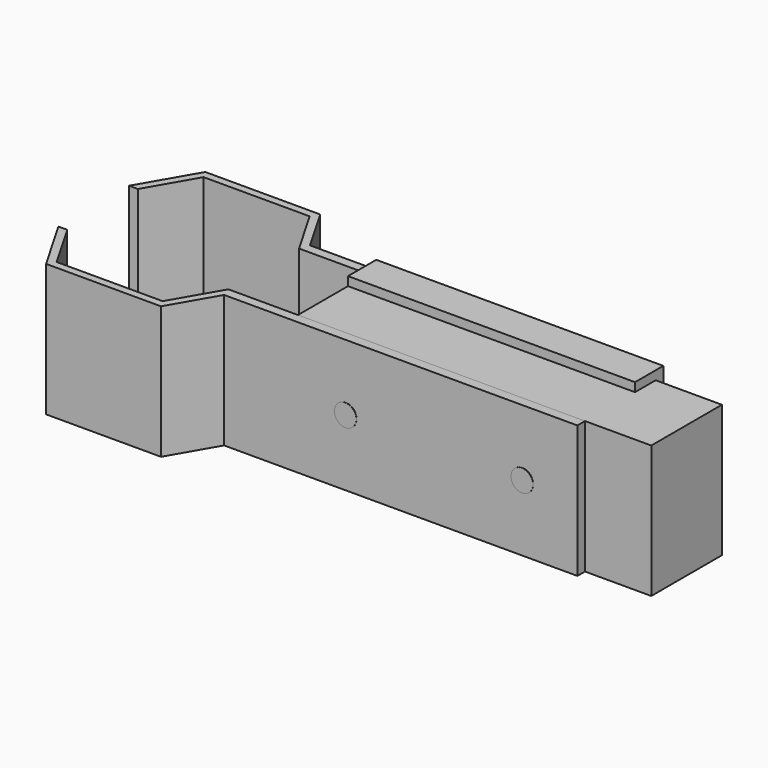
from build123d import *

# Parameters (mm, degrees)
F0_W      = 80
F0_H      = 20
F1_DEPTH  = 15
F3_DEPTH  = 50
F5_DEPTH  = 15
F7_W      = 80
F7_H      = 2.1551362713
F8_DEPTH  = 15
F9_W      = 14.0510366764
F9_H      = 20
F10_DEPTH = 20
F12_W     = 40
F12_H     = 20
F13_DEPTH = 15
F16_R     = 2.5
F17_DEPTH = 12.2
F19_W     = 65
F19_H     = 8
F20_DEPTH = 2
F22_W     = 65
F22_H     = 8
F23_DEPTH = 2
F25_R     = 2.5
F26_DEPTH = 1


# Not quite as in the source:
# - a feature of the source that left no trace in its solid (it failed there, or was rolled back) is left out


with BuildPart() as f1:
    # F0 (on Top) → F1 (new body, symmetric)
    with BuildSketch(Plane.XY):
        with Locations((40, 0)):
            Rectangle(F0_W, F0_H)
    extrude(amount=F1_DEPTH, both=True)


with BuildPart() as f3:
    # F2 (on Top) → F3 (new body, symmetric)
    with BuildSketch(Plane.XY):
        Polygon((-21.9911144009, -20.8), (-9.9822288017, 0), (-21.9911144009, 20.8), (-46.0088855991, 20.8), (-58.0177711983, 0), (-46.0088855991, -20.8), align=None)
    extrude(amount=F3_DEPTH, both=True)


with BuildPart() as f5:
    # F4 (on Top) → F5 (new body, symmetric)
    with BuildSketch(Plane.XY):
        Polygon((-20.9911144009, -22.5320508076), (-7.9822288017, 0), (-20.9911144009, 22.5320508076), (-47.0088855991, 22.5320508076), (-60.0177711983, 0), (-47.0088855991, -22.5320508076), align=None)
    extrude(amount=F5_DEPTH, both=True)

    # F6: cut F3
    add(f3.part, mode=Mode.SUBTRACT)

    # F7 (on Top) → F8, piece 2 (join, symmetric)
    with BuildSketch(Plane.XY):
        with Locations((25, -11.0775681357)):
            Rectangle(F7_W, F7_H)
    extrude(amount=F8_DEPTH, both=True)


with BuildPart() as f8:
    # F7 (on Top) → F8 (new body, symmetric)
    with BuildSketch(Plane.XY):
        with Locations((25, 11.0775681357)):
            Rectangle(F7_W, F7_H)
    extrude(amount=F8_DEPTH, both=True)

    # F19 (on offset) → F20 (join)
    with BuildSketch(Plane.XY.offset(15)):
        with Locations((32.5, 8.1551362713)):
            Rectangle(F19_W, F19_H)
    extrude(amount=F20_DEPTH)

    # F22 (on offset) → F23 (join)
    with BuildSketch(Plane(origin=(0, 0, -15), x_dir=(1, 0, 0), z_dir=(0, 0, -1))):
        with Locations((32.5, -8.1551362713)):
            Rectangle(F22_W, F22_H)
    extrude(amount=F23_DEPTH)


with BuildPart() as f10:
    # F9 (on Top) → F10 (new body, symmetric)
    with BuildSketch(Plane.XY):
        with Locations((-10.8901850181, 0)):
            Rectangle(F9_W, F9_H)
    extrude(amount=F10_DEPTH, both=True)


with BuildPart() as f5_1:
    add(f5.part)

    # F11: cut F10
    add(f10.part, mode=Mode.SUBTRACT)


with BuildPart() as f13:
    # F12 (on Top) → F13 (new body, symmetric)
    with BuildSketch(Plane.XY):
        with Locations((-50.3287625449, 0)):
            Rectangle(F12_W, F12_H)
    extrude(amount=F13_DEPTH, both=True)


with BuildPart() as f5_2:
    add(f5_1.part)

    # F14: cut F13
    add(f13.part, mode=Mode.SUBTRACT)

    # F16 (on Front) → F17 (join)
    with BuildSketch(Plane.XZ):
        with Locations((12.5, 0)):
            Circle(F16_R)
        with Locations((52.5, 0)):
            Circle(F16_R)
    extrude(amount=F17_DEPTH)


with BuildPart() as f8_1:
    add(f8.part)

    # F24: union F5
    add(f5_2.part)

    # F25 (on face) → F26 (join)
    with BuildSketch(Plane(origin=(0, 12.1551362713, 0), x_dir=(-1, 0, 0), z_dir=(0, 1, 0))):
        with Locations((-32.5, 0)):
            Circle(F25_R)
    extrude(amount=F26_DEPTH)


solid = Compound([f1.part, f8_1.part])
